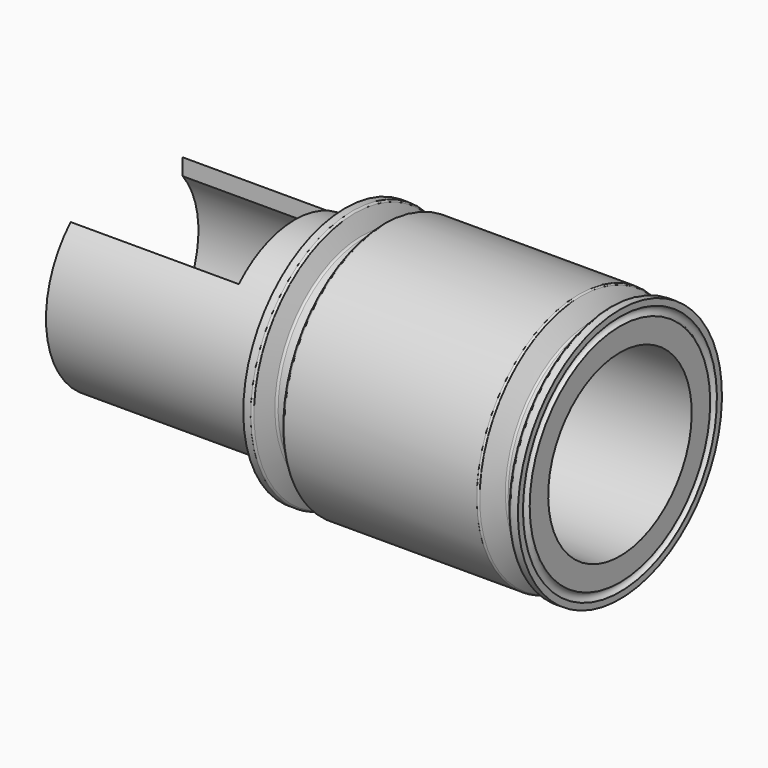
from build123d import *

# Parameters (mm, degrees)
F3_R        = 21.5
F4_DEPTH    = 25
F6_W        = 60
F6_H        = 50
F7_DEPTH    = 30
F8_T4_ANGLE = 73.3070095704
F8_T9_ANGLE = 73.3070095704


# Not quite as in the source:
# - a fillet or chamfer that OpenCascade refuses, or shapes differently, is made with other operations: its cross-section is extruded or revolved along the edge and cut away or added


with BuildPart() as f1:
    # F0 (on Front) → F1 (revolve)
    with BuildSketch(Plane.XZ):
        with BuildLine():
            Line((-176, 36), (-176, 32))
            Line((-176, 32), (0, 32))
            Line((0, 32), (0, 40.25))
            ThreePointArc((0, 40.25), (-1.5, 41.75), (0, 43.25))
            Line((0, 43.25), (0, 45.5))
            Line((0, 45.5), (-2.6398339694, 45.5))
            ThreePointArc((-2.6398339694, 45.5), (-3.0986951185, 45.3553216354), (-3.3915880661, 44.9736161147))
            Line((-3.3915880661, 44.9736161147), (-5.7199901792, 38.5763838853))
            ThreePointArc((-5.7199901792, 38.5763838853), (-6.0128831268, 38.1946783646), (-6.4717442759, 38.05))
            Line((-6.4717442759, 38.05), (-9.4496980299, 38.05))
            ThreePointArc((-9.4496980299, 38.05), (-9.8496980299, 38.157179677), (-10.142518353, 38.45))
            Line((-10.142518353, 38.45), (-13.9818976431, 45.1))
            ThreePointArc((-13.9818976431, 45.1), (-14.2747179661, 45.392820323), (-14.6747179661, 45.5))
            Line((-14.6747179661, 45.5), (-83.3252820339, 45.5))
            ThreePointArc((-83.3252820339, 45.5), (-83.7252820339, 45.392820323), (-84.0181023569, 45.1))
            Line((-84.0181023569, 45.1), (-87.857481647, 38.45))
            ThreePointArc((-87.857481647, 38.45), (-88.1503019701, 38.157179677), (-88.5503019701, 38.05))
            Line((-88.5503019701, 38.05), (-91.5282557241, 38.05))
            ThreePointArc((-91.5282557241, 38.05), (-91.9871168732, 38.1946783646), (-92.2800098208, 38.5763838853))
            Line((-92.2800098208, 38.5763838853), (-94.6084119339, 44.9736161147))
            ThreePointArc((-94.6084119339, 44.9736161147), (-94.9013048815, 45.3553216354), (-95.3601660306, 45.5))
            Line((-95.3601660306, 45.5), (-98, 45.5))
            Line((-98, 45.5), (-98, 43.25))
            ThreePointArc((-98, 43.25), (-96.5, 41.75), (-98, 40.25))
            Line((-98, 40.25), (-98, 36))
            Line((-98, 36), (-176, 36))
        make_face()
    revolve(axis=Axis((-38.3716828611, 0, 0), (-1, 0, 0)))

    # F3 (on offset) → F4 (cut)
    with BuildSketch(Plane.XY.offset(-45.5)):
        with Locations((-60, 0)):
            Circle(F3_R)
    extrude(amount=F4_DEPTH, mode=Mode.SUBTRACT)

    # F6 (on offset) → F7 (cut)
    with BuildSketch(Plane.XY.offset(45.5)):
        with Locations((-146, 0)):
            Rectangle(F6_W, F6_H)
    extrude(amount=-F7_DEPTH, mode=Mode.SUBTRACT)

    # F8: fillet of radius 5 on 2 edges, made by hand


with BuildPart() as f8_tool2:
    # F8_s3 → F8_t4 (revolve)
    with BuildSketch(Plane.XZ):
        with BuildLine():
            ThreePointArc((-111.1010205144, 32), (-114.2632981746, 33.1270166538), (-116, 36))
            Line((-116, 36), (-116, 32))
            Line((-116, 32), (-111.1010205144, 32))
        make_face()
    revolve(axis=Axis((-116, 0, 0), (1, 0, 0)), revolution_arc=F8_T4_ANGLE)

    split(bisect_by=Plane.XZ.offset(25), keep=Keep.BOTTOM)


with BuildPart() as f1_1:
    add(f1.part)

    # F8_t1: cut F8_tool2
    add(f8_tool2.part, mode=Mode.SUBTRACT)


with BuildPart() as f8_tool7:
    # F8_s8 → F8_t9 (revolve)
    with BuildSketch(Plane(origin=(0, 0, 0), x_dir=(1, 0, 0), z_dir=(0, 0.2872433376, -0.9578576434))):
        with BuildLine():
            ThreePointArc((-111.1010205144, -32), (-114.2632981746, -33.1270166538), (-116, -36))
            Line((-116, -36), (-116, -32))
            Line((-116, -32), (-111.1010205144, -32))
        make_face()
    revolve(axis=Axis((-116, 0, 0), (1, 0, 0)), revolution_arc=F8_T9_ANGLE)

    split(bisect_by=Plane.XZ.offset(-25), keep=Keep.TOP)


with BuildPart() as f1_2:
    add(f1_1.part)

    # F8_t6: cut F8_tool7
    add(f8_tool7.part, mode=Mode.SUBTRACT)


solid = f1_2.part
